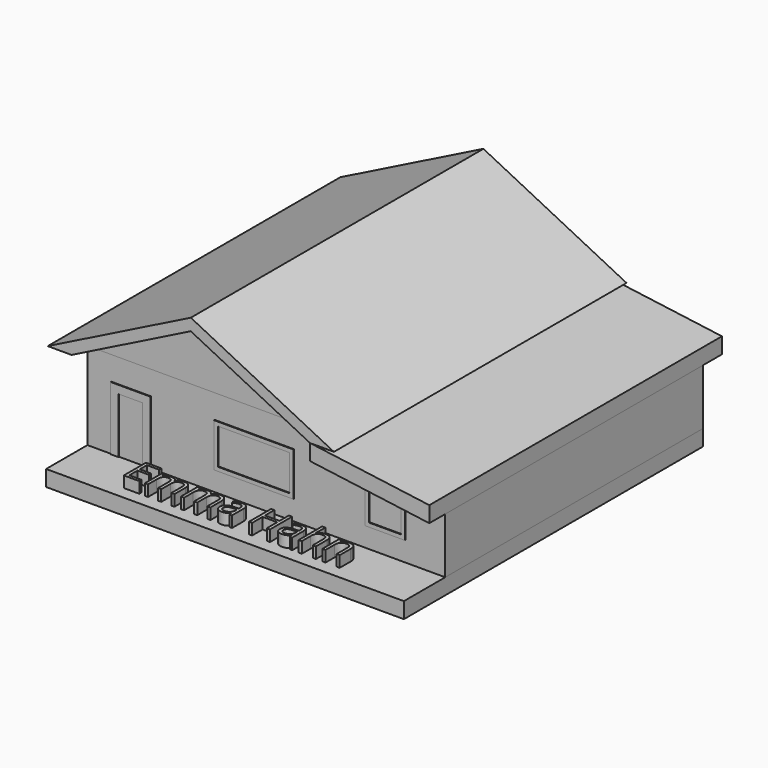
from build123d import *

# Parameters (mm, degrees)
F1_DEPTH      = 914.4
F1_DEPTH_BACK = 13106.4
F2_DEPTH      = 152.4
F2_DEPTH_BACK = 12192
F0_W          = 3048
F0_H          = 1676.4
F0_W_2        = 1524.0000335693
F0_H_2        = 1371.6
F0_W_3        = 2743.2
F0_W_4        = 1219.2
F0_H_3        = 1066.7999664307
F0_W_5        = 914.4
F0_H_4        = 2133.6
F3_DEPTH      = 152.4
F3_DEPTH_BACK = 12192
F4_DEPTH      = 2133.6
F4_DEPTH_BACK = 12192
F5_DEPTH      = 182.88
F5_DEPTH_BACK = 30.48
F6_TEXT_SIZE  = 1484.4716423088
F7_DEPTH      = 426.72
F8_W          = 2133.5999444962
F8_H          = 1523.9999444962
F8_W_2        = 1828.8
F8_H_2        = 1219.2
F9_DEPTH      = 152.4
F10_DEPTH     = 152.4


# Not quite as in the source:
# - Text() gives the source's letters only with a copy of the font that has no kerning and outlines rounded to 1/6400 em; it was checked with that copy


with BuildPart() as f1:
    # F0 (on Front) → F1 (new body, two sides)
    with BuildSketch(Plane.XZ) as f1_sk:
        Polygon((-5486.4, 0), (-4572, 0), (0, 2286), (0, 2743.2), align=None)
        Polygon((0, 2286), (4572, 0), (5486.4, 0), (0, 2743.2), align=None)
    extrude(amount=F1_DEPTH)
    extrude(f1_sk.sketch, amount=-F1_DEPTH_BACK)



with BuildPart() as f1b:
    # F0 (on Front) → F1, piece 2 (new body, two sides)
    with BuildSketch(Plane.XZ) as f1_2_sk:
        Polygon((9144, -609.6), (4572, 0), (4572, -609.6), (9144, -1219.2), align=None)
    extrude(amount=F1_DEPTH)
    extrude(f1_2_sk.sketch, amount=-F1_DEPTH_BACK)


with BuildPart() as f1_1:
    add(f1.part)

    add(f1b.part)  # F2 merges F1b
    # F0 (on Front) → F2 (join, two sides)
    with BuildSketch(Plane.XZ) as f2_sk:
        Polygon((0, 2286), (0, 0), (4572, 0), align=None)
        Polygon((-4572, 0), (0, 0), (0, 2286), align=None)
    extrude(amount=F2_DEPTH)
    extrude(f2_sk.sketch, amount=-F2_DEPTH_BACK)


with BuildPart() as f3:
    # F0 (on Front) → F3 (new body, two sides)
    with BuildSketch(Plane.XZ) as f3_sk:
        Polygon((4572, 0), (0, 0), (-4572, 0), (-4572, -3352.8), (-3657.6000034332, -3352.8), (-3657.6000034332, -914.3999965668), (-2133.5999965668, -914.3999965668), (-2133.5999965668, -3352.8), (4572, -3352.8), (4572, -609.6), align=None)
        with Locations((1828.8, -1752.6)):
            Rectangle(F0_W, F0_H, mode=Mode.SUBTRACT)
        Polygon((9144, -1219.2), (4572, -609.6), (4572, -3352.8), (9144, -3352.8), align=None)
        with Locations((6858.0000167847, -1905)):
            Rectangle(F0_W_2, F0_H_2, mode=Mode.SUBTRACT)
        with Locations((1828.8, -1752.6)):
            Rectangle(F0_W, F0_H)
        with Locations((1828.8, -1752.6)):
            Rectangle(F0_W_3, F0_H_2, mode=Mode.SUBTRACT)
        with Locations((1828.8, -1752.6)):
            Rectangle(F0_W_3, F0_H_2)
        with Locations((6858.0000167847, -1905)):
            Rectangle(F0_W_2, F0_H_2)
        with Locations((6858.0000167847, -1905)):
            Rectangle(F0_W_4, F0_H_3, mode=Mode.SUBTRACT)
        with Locations((-2895.6, -2286)):
            Rectangle(F0_W_5, F0_H_4)
        Polygon((-3657.6000034332, -914.3999965668), (-3657.6000034332, -3352.8), (-3352.8, -3352.8), (-3352.8, -1219.2), (-2438.4, -1219.2), (-2438.4, -3352.8), (-2133.5999965668, -3352.8), (-2133.5999965668, -914.3999965668), align=None)
        with Locations((6858.0000167847, -1905)):
            Rectangle(F0_W_4, F0_H_3)
    extrude(amount=F3_DEPTH)
    extrude(f3_sk.sketch, amount=-F3_DEPTH_BACK)

    # F0 (on Front) → F4 (join, two sides)
    with BuildSketch(Plane.XZ) as f4_sk:
        Polygon((-3657.6000034332, -3352.8), (-4572, -3352.8), (-4572, -3962.4), (4572, -3962.4), (4572, -3352.8), (-2133.5999965668, -3352.8), (-2438.4, -3352.8), (-3352.8, -3352.8), align=None)
        Polygon((9144, -3352.8), (4572, -3352.8), (4572, -3962.4), (9144.3004608154, -3962.4), align=None)
    extrude(amount=F4_DEPTH)
    extrude(f4_sk.sketch, amount=-F4_DEPTH_BACK)

    # F0 (on Front) → F5 (join, two sides)
    with BuildSketch(Plane.XZ) as f5_sk:
        Polygon((-3657.6000034332, -914.3999965668), (-3657.6000034332, -3352.8), (-3352.8, -3352.8), (-3352.8, -1219.2), (-2438.4, -1219.2), (-2438.4, -3352.8), (-2133.5999965668, -3352.8), (-2133.5999965668, -914.3999965668), align=None)
        with Locations((1828.8, -1752.6)):
            Rectangle(F0_W, F0_H)
        with Locations((1828.8, -1752.6)):
            Rectangle(F0_W_3, F0_H_2, mode=Mode.SUBTRACT)
        with Locations((6858.0000167847, -1905)):
            Rectangle(F0_W_2, F0_H_2)
        with Locations((6858.0000167847, -1905)):
            Rectangle(F0_W_4, F0_H_3, mode=Mode.SUBTRACT)
    extrude(amount=F5_DEPTH)
    extrude(f5_sk.sketch, amount=-F5_DEPTH_BACK)

    # F6 (on face) → F7 (join)
    with BuildSketch(Plane.XY.offset(-3352.8)):
        with Locations((-2126.0645389557, -1646.8697786331)):
            Text('Emma Hahn', F6_TEXT_SIZE, font='Open Sans', text_align=(TextAlign.LEFT, TextAlign.BOTTOM))
    extrude(amount=F7_DEPTH)

    # F8 (on face) → F9 (join)
    with BuildSketch(Plane(origin=(-4572, 0, 0), x_dir=(0, -1, 0), z_dir=(-1, 0, 0))):
        with Locations((-9601.2000277519, -1674.3086055756)):
            Rectangle(F8_W, F8_H)
        with Locations((-9601.2000277519, -1674.3086055756)):
            Rectangle(F8_W_2, F8_H_2, mode=Mode.SUBTRACT)
    extrude(amount=F9_DEPTH)

    # F8 (on face) → F10 (join)
    with BuildSketch(Plane(origin=(-4572, 0, 0), x_dir=(0, -1, 0), z_dir=(-1, 0, 0))):
        with Locations((-9601.2000277519, -1674.3086055756)):
            Rectangle(F8_W, F8_H)
        with Locations((-9601.2000277519, -1674.3086055756)):
            Rectangle(F8_W_2, F8_H_2, mode=Mode.SUBTRACT)
        with Locations((-2407.9199722481, -1674.3086055756)):
            Rectangle(F8_W, F8_H)
        with Locations((-2407.9199722481, -1674.3086055756)):
            Rectangle(F8_W_2, F8_H_2, mode=Mode.SUBTRACT)
    extrude(amount=F10_DEPTH)


solid = Compound([f1_1.part, f3.part])
